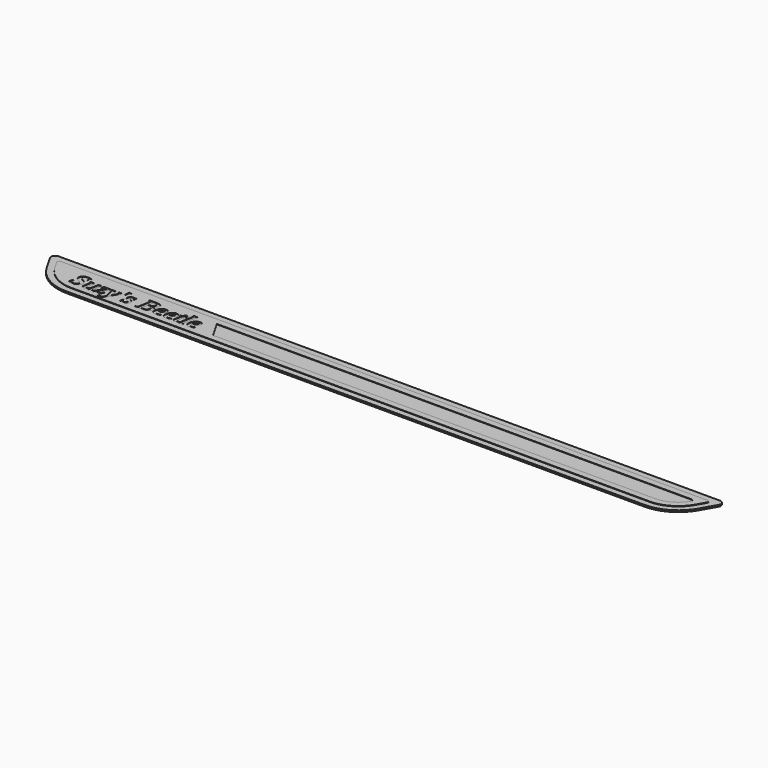
from build123d import *

# Parameters (mm, degrees)
F1_DEPTH     = 2
F3_DEPTH     = 0.5
F4_TEXT_SIZE = 27.7777777778
F5_DEPTH     = 0.5


# Not quite as in the source:
# - Text() gives the source's letters only with a copy of the font that has no kerning and outlines rounded to 1/6400 em; it was checked with that copy


with BuildPart() as f1:
    # F0 (on Top) → F1 (new body)
    with BuildSketch(Plane.XY):
        with BuildLine():
            Line((-340.9252271189, -25), (340.9252271189, -25))
            ThreePointArc((340.9252271189, -25), (365.9252271189, -18.3012701892), (384.2264973081, 0))
            Line((384.2264973081, 0), (394.3301270189, 17.5))
            ThreePointArc((394.3301270189, 17.5), (394.3301270189, 22.5), (390, 25))
            Line((390, 25), (-390, 25))
            ThreePointArc((-390, 25), (-394.3301270189, 22.5), (-394.3301270189, 17.5))
            Line((-394.3301270189, 17.5), (-384.2264973081, 0))
            ThreePointArc((-384.2264973081, 0), (-365.9252271189, -18.3012701892), (-340.9252271189, -25))
        make_face()
    extrude(amount=F1_DEPTH)


with BuildPart() as f3:
    # F2 (on face) → F3 (new body)
    with BuildSketch(Plane.XY.offset(2)):
        with BuildLine():
            ThreePointArc((340.9252271189, -17.5), (362.1752271189, -11.8060796608), (377.7313067797, 3.75))
            Line((377.7313067797, 3.75), (383.5048094716, 13.75))
            ThreePointArc((383.5048094716, 13.75), (383.5048094716, 16.25), (381.3397459622, 17.5))
            Line((381.3397459622, 17.5), (-381.3397459622, 17.5))
            ThreePointArc((-381.3397459622, 17.5), (-383.5048094716, 16.25), (-383.5048094716, 13.75))
            Line((-383.5048094716, 13.75), (-377.7313067797, 3.75))
            ThreePointArc((-377.7313067797, 3.75), (-362.1752271189, -11.8060796608), (-340.9252271189, -17.5))
            Line((-340.9252271189, -17.5), (340.9252271189, -17.5))
        make_face()
        with BuildLine():
            Line((-191.5470053838, 10), (368.3113549941, 10))
            ThreePointArc((368.3113549941, 10), (370.5040000424, 8.7009611535), (370.4179802153, 6.1538461538))
            ThreePointArc((370.4179802153, 6.1538461538), (357.7386832684, -5.6970306757), (340.9252271189, -10))
            Line((340.9252271189, -10), (-180, -10))
            Line((-180, -10), (-191.5470053838, 10))
        make_face(mode=Mode.SUBTRACT)
    extrude(amount=F3_DEPTH)

    # F4 (on face) → F5 (cut)
    with BuildSketch(Plane.XY.offset(2.5)):
        with Locations((-351.5885416667, -10)):
            Text("Suzy's Beetle", F4_TEXT_SIZE, font='Tinos', font_style=FontStyle.BOLDITALIC, text_align=(TextAlign.LEFT, TextAlign.BOTTOM))
    extrude(amount=-F5_DEPTH, mode=Mode.SUBTRACT)


solid = Compound([f1.part, f3.part])
